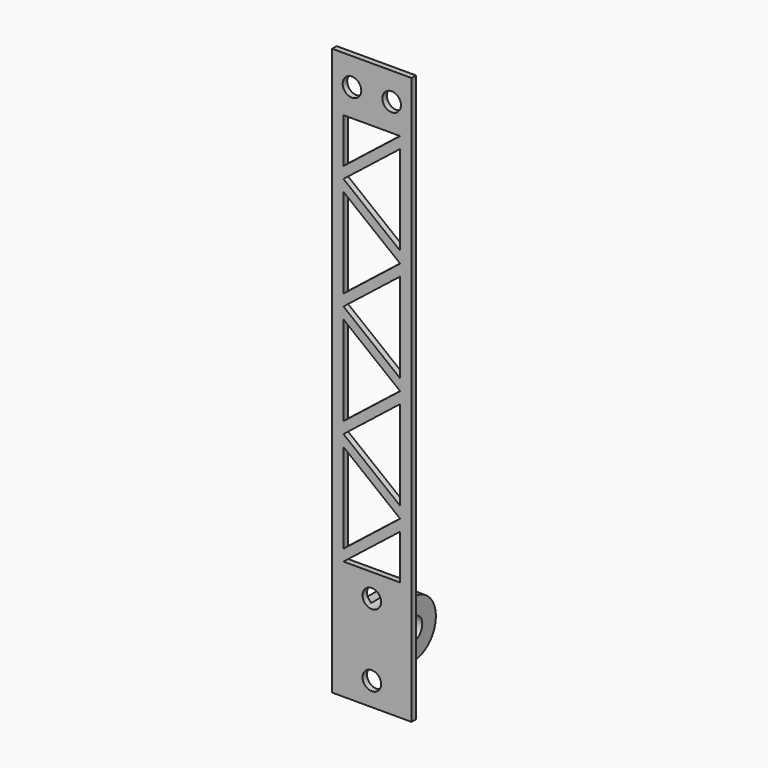
from build123d import *
from build123d import SkipClean  # not in build123d's __all__

# Parameters (mm, degrees)
F0_W     = 14
F0_H     = 100
F0_R     = 1.64
F1_DEPTH = 1
F2_DEPTH = 10
F3_R     = 2
F4_DEPTH = 9.501


# Not quite as in the source:
# - after a boolean that leaves OpenCascade's solid faulty, fix() repairs it
# - a feature names something its author has since deleted; it is built from what else it names


with BuildPart() as f1:
    # F0 (on Front) → F1 (new body)
    with BuildSketch(Plane.XZ):
        Rectangle(F0_W, F0_H)
        with BuildLine():
            Line((-2.5, -44.5), (-2.5, -34.5))
            Line((-2.5, -34.5), (-0.8938540149, -34.5))
            ThreePointArc((-0.8938540149, -34.5), (-0.7822018331, -31.6835561779), (1.64, -33.125))
            ThreePointArc((1.64, -33.125), (1.4414438221, -33.9072018331), (0.8938540149, -34.5))
            Line((0.8938540149, -34.5), (2.5, -34.5))
            Line((2.5, -34.5), (2.5, -44.5))
            Line((2.5, -44.5), (0.8938540149, -44.5))
            ThreePointArc((0.8938540149, -44.5), (1.4414438221, -45.0927981669), (1.64, -45.875))
            ThreePointArc((1.64, -45.875), (-0.7822018331, -47.3164438221), (-0.8938540149, -44.5))
            Line((-0.8938540149, -44.5), (-2.5, -44.5))
        make_face(mode=Mode.SUBTRACT)
        Polygon((5, -21.096), (5, -29), (-5, -29), align=None, mode=Mode.SUBTRACT)
        Polygon((5, -19.096), (-5, -27), (-5, -11.192), align=None, mode=Mode.SUBTRACT)
        Polygon((5, -17.096), (-5, -9.192), (5, -1.288), align=None, mode=Mode.SUBTRACT)
        with Locations((-3.5, 45.167)):
            Circle(F0_R, mode=Mode.SUBTRACT)
        Polygon((-5, -7.19), (-5, 8.618), (5, 0.714), align=None, mode=Mode.SUBTRACT)
        Polygon((5, 18.522), (5, 2.714), (-5, 10.618), align=None, mode=Mode.SUBTRACT)
        Polygon((-5, 12.62), (-5, 28.428), (5, 20.524), align=None, mode=Mode.SUBTRACT)
        Polygon((5, 38.332), (5, 22.524), (-5, 30.428), align=None, mode=Mode.SUBTRACT)
        Polygon((5, 40.334), (-5, 32.43), (-5, 40.334), align=None, mode=Mode.SUBTRACT)
        with Locations((3.5, 45.167)):
            Circle(F0_R, mode=Mode.SUBTRACT)
        with BuildLine():
            Line((-0.8938540149, -34.5), (-2.5, -34.5))
            Line((-2.5, -34.5), (-2.5, -44.5))
            Line((-2.5, -44.5), (-0.8938540149, -44.5))
            ThreePointArc((-0.8938540149, -44.5), (0, -44.235), (0.8938540149, -44.5))
            Line((0.8938540149, -44.5), (2.5, -44.5))
            Line((2.5, -44.5), (2.5, -34.5))
            Line((2.5, -34.5), (0.8938540149, -34.5))
            ThreePointArc((0.8938540149, -34.5), (0, -34.765), (-0.8938540149, -34.5))
        make_face()
    extrude(amount=F1_DEPTH)

    # F0 (on Front) → F2 (join)
    with BuildSketch(Plane.XZ):
        with BuildLine():
            Line((-0.8938540149, -34.5), (-2.5, -34.5))
            Line((-2.5, -34.5), (-2.5, -44.5))
            Line((-2.5, -44.5), (-0.8938540149, -44.5))
            ThreePointArc((-0.8938540149, -44.5), (0, -44.235), (0.8938540149, -44.5))
            Line((0.8938540149, -44.5), (2.5, -44.5))
            Line((2.5, -44.5), (2.5, -34.5))
            Line((2.5, -34.5), (0.8938540149, -34.5))
            ThreePointArc((0.8938540149, -34.5), (0, -34.765), (-0.8938540149, -34.5))
        make_face()
    with SkipClean():  # cleaning this boolean's faces spoils the solid; the shape is the same uncleaned
        extrude(amount=-F2_DEPTH)

    # F3 (on face) → F4 (cut, through all)
    with BuildSketch(Plane.YZ.offset(2.5)):
        with BuildLine():
            Line((5, -44.5), (10, -44.5))
            Line((10, -44.5), (10, -39.5))
            ThreePointArc((10, -39.5), (8.5355339059, -43.0355339059), (5, -44.5))
        make_face()
        with Locations((5, -39.5)):
            Circle(F3_R)
        with BuildLine():
            ThreePointArc((5, -34.5), (8.5355339059, -35.9644660941), (10, -39.5))
            Line((10, -39.5), (10, -34.5))
            Line((10, -34.5), (5, -34.5))
        make_face()
    extrude(amount=-F4_DEPTH, mode=Mode.SUBTRACT)

    add(f1.part.fix(), mode=Mode.REPLACE)


solid = f1.part
